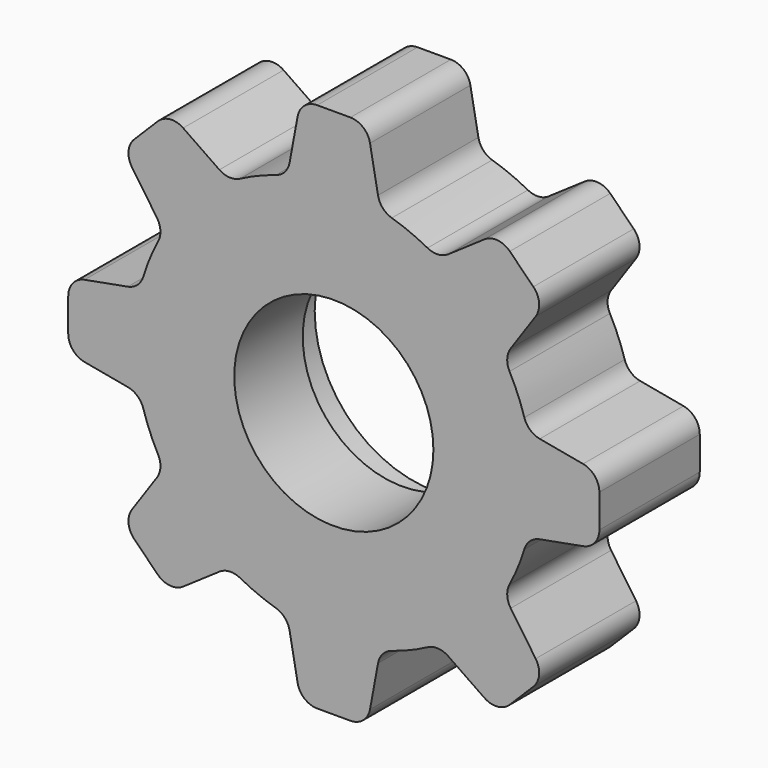
from build123d import *

# Parameters (mm, degrees)
F0_R            = 2.54
F0_R_2          = 1.27
F1_DEPTH        = 1.6002
F3_DEPTH        = 1.6002
F3_COPIES_COUNT = 8
F5_R            = 0.254
F6_R            = 1.524
F7_DEPTH        = 0.508


# Not quite as in the source:
# - a pattern or mirror of a feature is missing from the dataset's text; its kind, count and spacing are read off the source's solid


with BuildPart() as f1:
    # F0 (on Front) → F1 (new body)
    with BuildSketch(Plane.XZ):
        Circle(F0_R)
        Circle(F0_R_2, mode=Mode.SUBTRACT)
    extrude(amount=F1_DEPTH)

    # F2 (on face) → F3 (join, through all)
    with BuildSketch(Plane.XZ.offset(1.6002)):
        Polygon((0.4233333333, 3.3866666667), (-0.4233333333, 3.3866666667), (-0.5926666667, 2.4698878967), (0.5926666667, 2.4698878967), align=None)
    f3 = extrude(amount=-F3_DEPTH)

    # F3_copies: F3 ×8 about axis
    f3_copies_axis = Axis((0, 0, 0), (0, 1, 0))
    for i in range(1, F3_COPIES_COUNT):
        add(f3.rotate(f3_copies_axis, i * 360 / F3_COPIES_COUNT))

    # F5
    f5_edges = [f1.edges().sort_by_distance(p)[0] for p in [
        (-0.423333, -0.8001, 3.386667),
        (-0.592667, -0.8001, 2.469888),
        (0.423333, -0.8001, 3.386667),
        (0.592667, -0.8001, 2.469888),
        (-1.327396, -0.8001, 2.165553),
        (-2.095393, -0.8001, 2.694077),
        (2.165553, -0.8001, 1.327396),
        (2.694077, -0.8001, 2.095393),
        (2.469888, -0.8001, 0.592667),
        (3.386667, -0.8001, 0.423333),
        (3.386667, -0.8001, -0.423333),
        (2.469888, -0.8001, -0.592667),
        (2.165553, -0.8001, -1.327396),
        (2.694077, -0.8001, -2.095393),
        (2.095393, -0.8001, -2.694077),
        (1.327396, -0.8001, -2.165553),
        (0.592667, -0.8001, -2.469888),
        (0.423333, -0.8001, -3.386667),
        (-0.423333, -0.8001, -3.386667),
        (-0.592667, -0.8001, -2.469888),
        (-1.327396, -0.8001, -2.165553),
        (-2.095393, -0.8001, -2.694077),
        (-2.694077, -0.8001, -2.095393),
        (-2.165553, -0.8001, -1.327396),
        (-2.469888, -0.8001, -0.592667),
        (-3.386667, -0.8001, -0.423333),
        (-3.386667, -0.8001, 0.423333),
        (-2.469888, -0.8001, 0.592667),
        (-2.165553, -0.8001, 1.327396),
        (1.327396, -0.8001, 2.165553),
        (2.095393, -0.8001, 2.694077),
        (-2.694077, -0.8001, 2.095393),
    ]]
    fillet(f5_edges, radius=F5_R)

    # F6 (on face) → F7 (cut)
    with BuildSketch(Plane(origin=(0, 0, 0), x_dir=(-1, 0, 0), z_dir=(0, 1, 0))):
        Circle(F6_R)
    extrude(amount=-F7_DEPTH, mode=Mode.SUBTRACT)


solid = f1.part
